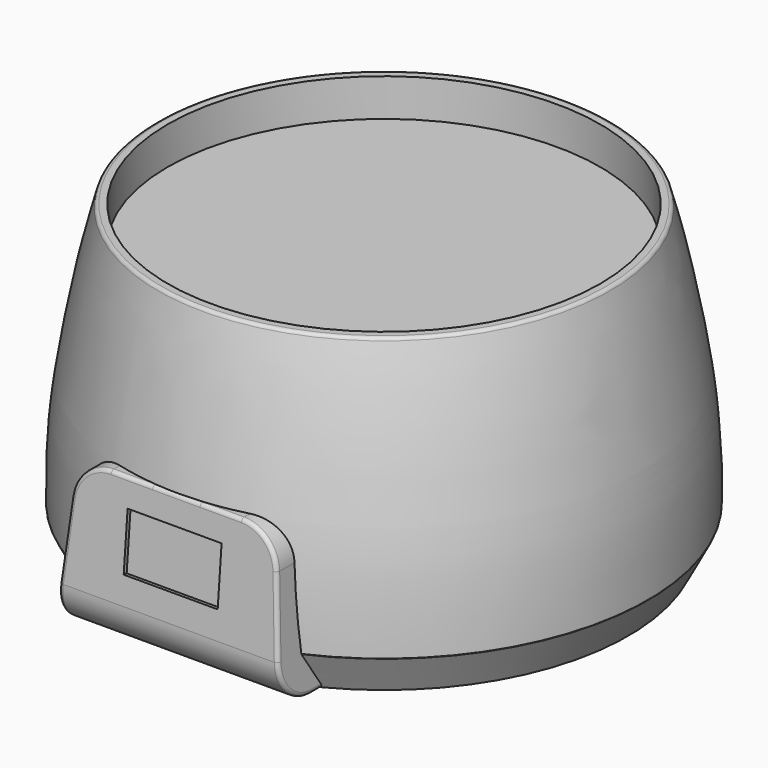
from build123d import *

# Parameters (mm, degrees)
F2_W      = 30
F2_H      = 15
F3_DEPTH  = 40
F3_TAPER  = 5
F4_R      = 10
F5_R      = 10
F6_R      = 57.5
F7_DEPTH  = 10
F8_R      = 1
F9_W      = 12.5
F9_H      = 15
F10_DEPTH = 1
F11_R     = 1


with BuildPart() as f1:
    # F0 (on Front) → F1 (revolve)
    with BuildSketch(Plane.XZ):
        with BuildLine():
            Line((-65, 0), (0, 0))
            Line((0, 0), (0, 80))
            Line((0, 80), (-60, 80))
            add(Edge.make_bspline(
                [(-70.1933311222, 10.0818746543), (-70.63559014, 24.2740495561), (-67.5765539829, 48.5172165288), (-62.8462281818, 69.8161359517), (-60, 80)],
                knots=[0.0010082703, 0.0010082703, 0.0010082703, 0.0010082703, 0.5254339339, 1, 1, 1, 1], degree=3))
            Line((-70.1933311222, 10.0818746543), (-69.9069664697, 10.0827200882))
            Line((-69.9069664697, 10.0827200882), (-69.9069664697, 10))
            Line((-69.9069664697, 10), (-70.190757513, 10))
            Line((-70.190757513, 10), (-65, 0))
        make_face()
    revolve(axis=Axis((0, 0, 40), (0, 0, 1)))

    # F2 (on Top) → F3 (join)
    with BuildSketch(Plane.XY):
        with Locations((15, -57.5)):
            Rectangle(F2_W, F2_H)
        with Locations((-15, -57.5)):
            Rectangle(F2_W, F2_H)
        Polygon((30, -65), (0, -65), (-30, -65), (-30, -72.5), (30, -72.5), align=None)
    extrude(amount=F3_DEPTH, taper=F3_TAPER)

    # F4
    f4_edges = [f1.edges().sort_by_distance(p)[0] for p in [
        (-26.500453, -66.016212, 40),
        (26.500453, -66.016212, 40),
    ]]
    fillet(f4_edges, radius=F4_R)

    # F5
    f5_edges = [f1.edges().sort_by_distance(p)[0] for p in [
        (0, -72.5, 0),
    ]]
    fillet(f5_edges, radius=F5_R)

    # F6 (on face) → F7 (cut)
    with BuildSketch(Plane.XY.offset(80)):
        Circle(F6_R)
    extrude(amount=-F7_DEPTH, mode=Mode.SUBTRACT)

    # F8
    f8_edges = [f1.edges().sort_by_distance(p)[0] for p in [
        (60, 0, 80),
    ]]
    fillet(f8_edges, radius=F8_R)

    # F9 (on face) → F10 (cut)
    with BuildSketch(Plane(origin=(0, -71.9492810467, 6.2947464404), x_dir=(1, 0, 0), z_dir=(0, -0.9961946981, 0.0871557427))):
        with Locations((6.25, 19.214147907)):
            Rectangle(F9_W, F9_H)
        with Locations((-6.25, 19.214147907)):
            Rectangle(F9_W, F9_H)
    extrude(amount=-F10_DEPTH, mode=Mode.SUBTRACT)

    # F11
    f11_edges = [f1.edges().sort_by_distance(p)[0] for p in [
        (-29.715512, -68.966657, 3.25171),
        (0, -71.548862, 10.871557),
        (0, -61.586915, 0),
        (29.715512, -68.966657, 3.25171),
        (28.173975, -70.673975, 20.871557),
        (30, -59.624864, 0),
        (24.093044, -69.230306, 37.372773),
        (-28.173975, -70.673975, 20.871557),
        (-30, -59.624864, 0),
        (-24.093044, -69.230306, 37.372773),
    ]]
    fillet(f11_edges, radius=F11_R)


solid = f1.part
